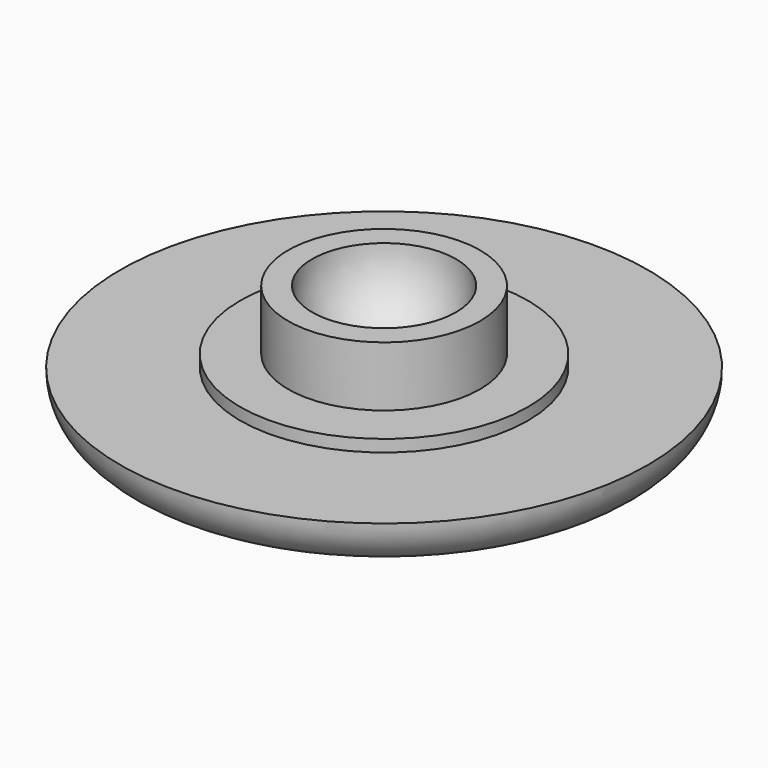
from build123d import *

# Parameters (mm, degrees)
F0_R      = 11
F1_DEPTH  = 2
F2_R      = 4
F3_DEPTH  = 3
F4_R      = 1.99999
F6_DEPTH  = 1
F8_R      = 3
F9_DEPTH  = 3
F10_R     = 2.99999
F11_R     = 6
F11_R_2   = 4
F12_DEPTH = 0.5


# Not quite as in the source:
# - a fillet or chamfer is up to 0.001 mm smaller than in the source, because OpenCascade refuses the exact size


with BuildPart() as f1:
    # F0 (on Top) → F1 (new body)
    with BuildSketch(Plane.XY):
        Circle(F0_R)
    extrude(amount=F1_DEPTH)

    # F2 (on face) → F3 (join)
    with BuildSketch(Plane.XY.offset(2)):
        Circle(F2_R)
    extrude(amount=F3_DEPTH)

    # F4 (radius 2 in the source; OpenCascade refuses exactly that, so slightly less here)
    f4_edges = [f1.edges().sort_by_distance(p)[0] for p in [
        (-11, 0, 0),
    ]]
    fillet(f4_edges, radius=F4_R)


with BuildPart() as f6:
    # F5 (on face) → F6 (new body)
    with BuildSketch(Plane(origin=(0, 0, 0), x_dir=(1, 0, 0), z_dir=(0, 0, -1))):
        with BuildLine():
            Line((-1.8928718055, -3.9824442938), (-0.9834596422, -7.5))
            Line((-0.9834596422, -7.5), (-0.4831294937, -4.1163032874))
            Line((-0.4831294937, -4.1163032874), (0, -4.1163032874))
            Line((0, -4.1163032874), (0, -1.9741227152))
            Line((0, -1.9741227152), (0.4605528779, -1.9741227152))
            Line((0.4605528779, -1.9741227152), (0.7225455958, 0.177173526))
            add(Edge.make_bspline(
                [(0.7225455958, 0.177173526), (0.7762262629, 0.2281189128), (0.8502513972, 0.379098319), (0.9568493801, 0.5825831672), (1.3882358596, 0.2713520899), (2.2706158575, 0.325109657), (2.9606627237, 0.5466543673), (3.1425092039, 1.1600376151), (3.6988276955, 0.9771075427), (4.3323473067, 1.21148059), (4.7251701582, 1.5841194333), (4.902445248, 2.0476494201), (4.5390546862, 2.3571166495), (4.868610307, 2.5728562245), (4.9005730312, 2.9881043818), (4.5078459511, 3.402767623), (4.1299512308, 3.3725223179), (4.1449199962, 3.7139472996), (3.7892118892, 4.0463374379), (3.2572627056, 4.1880335908), (2.7334793793, 4.2820261048), (2.1618953926, 3.897074129), (2.0720441471, 4.2415005639), (1.8459876198, 4.3387790504), (1.7167479964, 4.3746663272)],
                knots=[0, 0, 0, 0, 0.034315087, 0.0622229844, 0.1073020773, 0.1732684996, 0.2311308228, 0.279673902, 0.3272413623, 0.3836308507, 0.4348403206, 0.480326059, 0.5210456198, 0.5580673996, 0.6004997328, 0.6509122273, 0.6886586533, 0.7237040981, 0.7704572796, 0.821840504, 0.8731203646, 0.9242640946, 0.9576988474, 1, 1, 1, 1], degree=3))
            Line((1.7167479964, 4.3746663272), (1.7167479964, 6.2843358159))
            Line((1.7167479964, 6.2843358159), (-0.2752703829, 6.2843358159))
            Line((-0.2752703829, 6.2843358159), (-0.2752703829, 6.894516015))
            ThreePointArc((-0.2752703829, 6.894516015), (-0.4272640848, 7.5), (-0.5792577867, 6.894516015))
            Line((-0.5792577867, 6.894516015), (-0.5792577867, 6.2657745569))
            Line((-0.5792577867, 6.2657745569), (-2.6237959974, 6.2657745569))
            Line((-2.6237959974, 6.2657745569), (-2.6237959974, 4.3746663272))
            add(Edge.make_bspline(
                [(-2.6237959974, 4.3746663272), (-2.7796377607, 4.370777365), (-3.1414168436, 4.3183073448), (-4.073810314, 3.973406918), (-4.1413287087, 3.333735406), (-4.4619695731, 3.4550470658), (-4.8678120533, 3.3719150759), (-5.2219971301, 3.2049126023), (-5.4357633862, 2.9548787394), (-5.44929439, 2.6100254951), (-5.106905436, 2.4150215688), (-5.1288996618, 2.1963283303), (-5.3237832819, 2.0663564119), (-5.3964938936, 1.9264425574), (-5.4313375817, 1.5960952954), (-5.0652612539, 1.2757646634), (-4.6345917016, 1.2740107743), (-4.5809776708, 1.0145212389), (-4.1196007189, 0.7563932071), (-3.3948718138, 0.3896693064), (-2.2669242123, 0.6015313813), (-2.0057648306, 0.5739172824), (-1.9676401478, 0.4131318116), (-1.7577845477, 0.2956896244), (-1.6236169031, 0.2206049394)],
                knots=[0, 0, 0, 0, 0.0536267868, 0.125501705, 0.176884892, 0.2130500311, 0.2609244015, 0.3072661614, 0.3484970374, 0.388773427, 0.4324778226, 0.463109394, 0.4976120146, 0.5266797454, 0.5667035162, 0.6165113557, 0.6621433152, 0.6955544981, 0.7468759924, 0.8151348745, 0.8935257992, 0.9273075254, 0.9535099497, 1, 1, 1, 1], degree=3))
            Line((-1.6236169031, 0.2206049394), (-1.0462932987, -1.9002375193))
            Line((-1.0462932987, -1.9002375193), (-1.8196863821, -1.9002375193))
            Line((-1.8196863821, -1.9002375193), (-1.2898070272, -3.9824442938))
            Line((-1.2898070272, -3.9824442938), (-1.8928718055, -3.9824442938))
        make_face()
    extrude(amount=-F6_DEPTH)


with BuildPart() as f1_1:
    add(f1.part)

    # F7: cut F6
    add(f6.part, mode=Mode.SUBTRACT)

    # F8 (on face) → F9 (cut, through all)
    with BuildSketch(Plane.XY.offset(5)):
        Circle(F8_R)
    extrude(amount=-F9_DEPTH, mode=Mode.SUBTRACT)

    # F10 (radius 3 in the source; OpenCascade refuses exactly that, so slightly less here)
    f10_edges = [f1_1.edges().sort_by_distance(p)[0] for p in [
        (-3, 0, 2),
    ]]
    fillet(f10_edges, radius=F10_R)

    # F11 (on face) → F12 (join)
    with BuildSketch(Plane.XY.offset(2)):
        Circle(F11_R)
        Circle(F11_R_2, mode=Mode.SUBTRACT)
    extrude(amount=F12_DEPTH)


solid = Compound([f6.part, f1_1.part])
